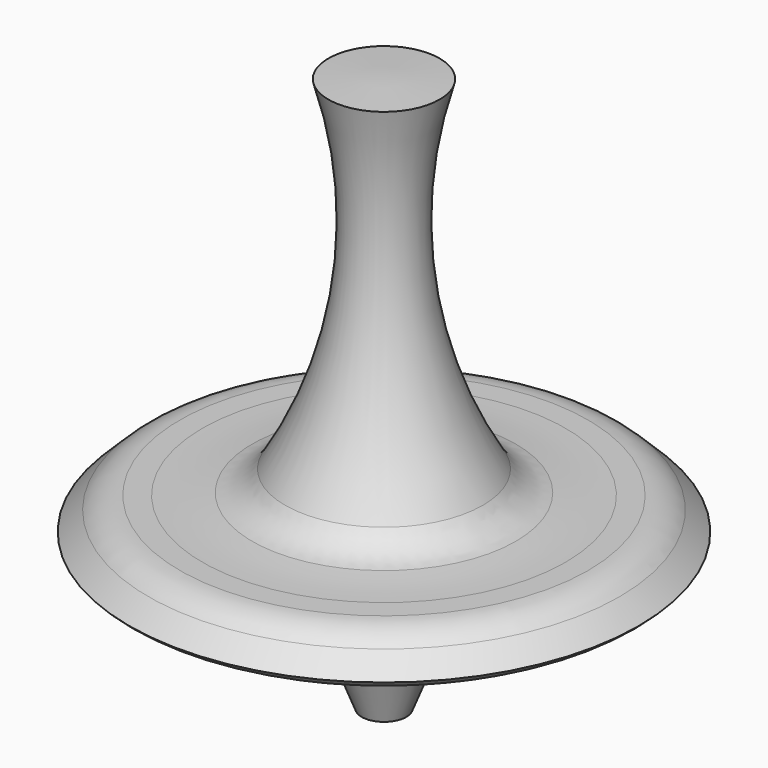
from build123d import *

# Parameters (mm, degrees)
F2_DEPTH = 12.7
F3_R     = 5.08
F5_R     = 5.08
F6_R     = 5.08


# Not quite as in the source:
# - a fillet or chamfer that OpenCascade refuses, or shapes differently, is made with other operations: its cross-section is extruded or revolved along the edge and cut away or added


with BuildPart() as f1:
    # F0 (on Front) → F1 (revolve)
    with BuildSketch(Plane.XZ):
        with BuildLine():
            Line((6.3432058776, 63.206334895), (0, 63.5))
            Line((0, 63.5), (0, 0))
            Line((0, 0), (2.5480911136, 0))
            Line((2.5480911136, 0), (6.6250329837, 10.4471649975))
            Line((6.6250329837, 10.4471649975), (10.9556252941, 16.1543861032))
            Line((10.9556252941, 16.1543861032), (30.48, 16.1543861032))
            Line((30.48, 16.1543861032), (30.4299078499, 21.4240159839))
            Line((30.4299078499, 21.4240159839), (20.699405237, 21.4240159839))
            ThreePointArc((20.699405237, 21.4240159839), (16.6336106625, 21.5337881018), (12.597086859, 22.0329985023))
            ThreePointArc((12.597086859, 22.0329985023), (4.7528583484, 41.9031506128), (6.3432058776, 63.206334895))
        make_face()
    revolve(axis=Axis((0, 0, 31.75), (0, 0, -1)))

    # F2 (cut): a face of the model
    f2_faces = [f1.faces().sort_by_distance(p)[0] for p in [
        (0, 0, 0),
    ]]
    extrude(f2_faces, amount=-F2_DEPTH, mode=Mode.SUBTRACT)

    # F3
    f3_edges = [f1.edges().sort_by_distance(p)[0] for p in [
        (-10.955625, 0, 16.154386),
        (-30.48, 0, 16.154386),
    ]]
    fillet(f3_edges, radius=F3_R)

    # F4: chamfer of 5.08 on 1 edges, made by hand

    # F4_s1 → F4_t2 (revolve, cut)
    with BuildSketch(Plane.XZ):
        Polygon((30.478195231, 16.3442454843), (25.3499078499, 21.4240159839), (30.4299078499, 21.4240159839), align=None)
    revolve(axis=Axis((0, 0, 21.4240159839), (0, 0, -1)), mode=Mode.SUBTRACT)

    # F5
    f5_edges = [f1.edges().sort_by_distance(p)[0] for p in [
        (-20.699405, 0, 21.424016),
        (-12.597087, 0, 22.032999),
        (16.633611, 0, 21.533788),
    ]]
    fillet(f5_edges, radius=F5_R)

    # F6
    f6_edges = [f1.edges().sort_by_distance(p)[0] for p in [
        (-25.349908, 0, 21.424016),
        (-20.699405, 0, 21.424016),
    ]]
    fillet(f6_edges, radius=F6_R)


solid = f1.part
